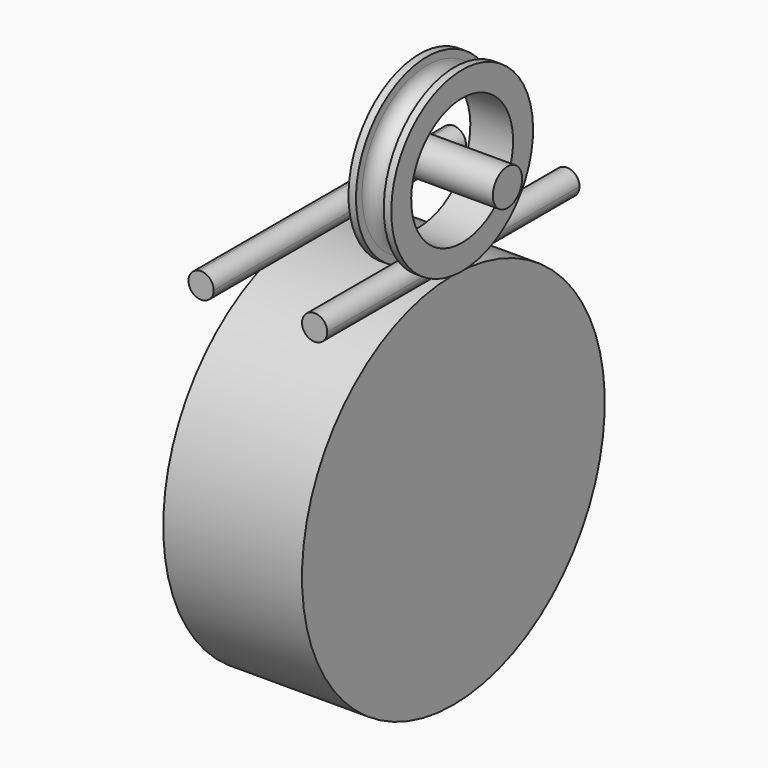
from build123d import *

# Parameters (mm, degrees)
F3_DEPTH = 12.5
F1_W     = 3.390828
F1_H     = 1.45


with BuildPart() as f3:
    # F2 (on Front) → F3 (new body, symmetric)
    with BuildSketch(Plane.XZ):
        with BuildLine():
            ThreePointArc((5.189161, -0.724608), (5.419011, -0.394233), (5.5, 0))
            ThreePointArc((5.5, 0), (4.5, 1), (3.5, 0))
            ThreePointArc((3.5, 0), (3.580989, -0.394233), (3.810839, -0.724608))
            Line((3.810839, -0.724608), (5.189161, -0.724608))
        make_face()
        with BuildLine():
            ThreePointArc((3.810839, -0.724608), (4.5, -1), (5.189161, -0.724608))
            Line((5.189161, -0.724608), (3.810839, -0.724608))
        make_face()
    extrude(amount=F3_DEPTH, both=True)


with BuildPart() as f3b:
    # F2 (on Front) → F3, piece 2 (new body, symmetric)
    with BuildSketch(Plane.XZ):
        with BuildLine():
            Line((-4.67896, -0.655514), (-4.67896, 0.983856))
            ThreePointArc((-4.67896, 0.983856), (-4.944948, 0.895556), (-5.175988, 0.736913))
            Line((-5.175988, 0.736913), (-5.175988, -0.655514))
            Line((-5.175988, -0.655514), (-4.67896, -0.655514))
        make_face()
        with BuildLine():
            ThreePointArc((-5.175988, 0.736913), (-4.9025, -0.91542), (-3.5, 0))
            ThreePointArc((-3.5, 0), (-3.859282, 0.767776), (-4.67896, 0.983856))
            Line((-4.67896, 0.983856), (-4.67896, -0.655514))
            Line((-4.67896, -0.655514), (-5.175988, -0.655514))
            Line((-5.175988, -0.655514), (-5.175988, 0.736913))
        make_face()
    extrude(amount=F3_DEPTH, both=True)


with BuildPart() as f4:
    # F1 (on Front) → F4 (revolve)
    with BuildSketch(Plane.XZ):
        with BuildLine():
            Line((2.804586, -0.6), (3.4, -0.6))
            Line((3.4, -0.6), (3.4, 0))
            ThreePointArc((3.4, 0), (4.5, 1.1), (5.6, 0))
            Line((5.6, 0), (5.6, -0.6))
            Line((5.6, -0.6), (6.195414, -0.6))
            Line((6.195414, -0.6), (6.195414, 1.376235))
            Line((6.195414, 1.376235), (4.5, 1.376235))
            Line((4.5, 1.376235), (2.804586, 1.376235))
            Line((2.804586, 1.376235), (2.804586, -0.6))
        make_face()
    revolve(axis=Axis((4.5, 0, 6.426235), (1, 0, 0)))


with BuildPart() as f4b:
    # F1 (on Front) → F4, piece 2 (revolve)
    with BuildSketch(Plane.XZ):
        with Locations((4.5, 5.701235)):
            Rectangle(F1_W, F1_H)
        Polygon((6.195414, 6.426235), (6.195414, 4.976235), (6.795414, 4.976235), (9.787117, 4.976235), (9.787117, 6.426235), align=None)
    revolve(axis=Axis((4.5, 0, 6.426235), (1, 0, 0)))


with BuildPart() as f5:
    # F1 (on Front) → F5 (revolve)
    with BuildSketch(Plane.XZ):
        Polygon((4.5, -1.1), (-5.5, -1.1), (-5.5, -16.1), (5.5, -16.1), (5.5, -1.1), align=None)
    revolve(axis=Axis((0, 0, -16.1), (1, 0, 0)))


solid = Compound([f3.part, f3b.part, f4.part, f4b.part, f5.part])
